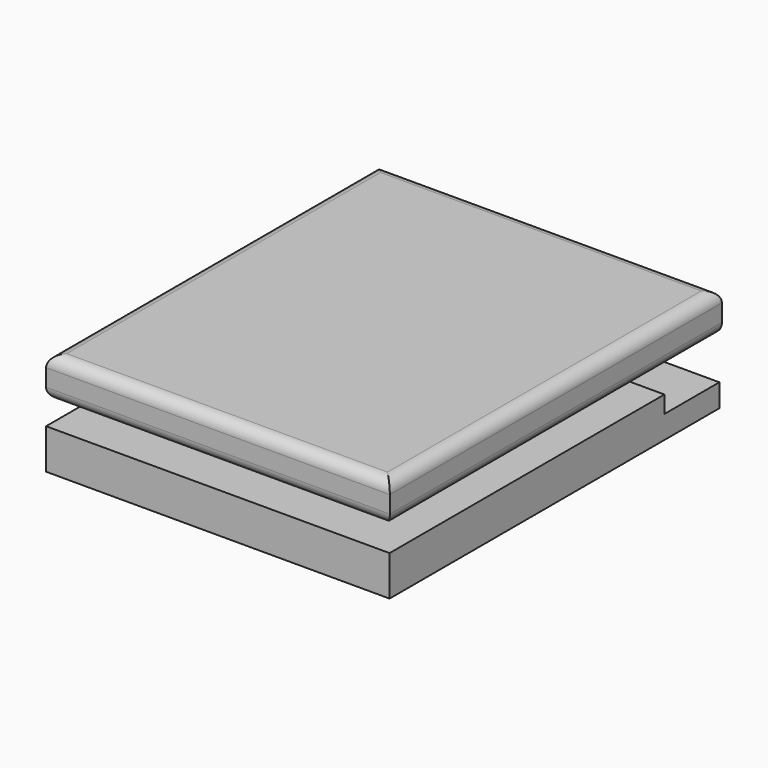
from build123d import *

# Parameters (mm, degrees)
F0_W        = 30
F0_H        = 30
F1_DEPTH    = 1.5
F2_W        = 15
F2_H        = 18.3394747698
F3_DEPTH    = 2
F4_W        = 30
F4_H        = 36
F5_DEPTH    = 2
F6_W        = 30.0186313689
F6_H        = 36.2569130957
F7_DEPTH    = 3.5
F8_T1_DEPTH = 15
F8_T3_DEPTH = 41.2569130957
F8_T5_DEPTH = 35.0186313689


# Not quite as in the source:
# - a fillet or chamfer that OpenCascade refuses, or shapes differently, is made with other operations: its cross-section is extruded or revolved along the edge and cut away or added


with BuildPart() as f1:
    # F0 (on Top) → F1 (new body)
    with BuildSketch(Plane.XY):
        with Locations((15, 15)):
            Rectangle(F0_W, F0_H)
    extrude(amount=F1_DEPTH)

    # F2 (on face) → F3 (join)
    with BuildSketch(Plane.XY.offset(1.5)):
        with Locations((14.8406922431, 27.8302626151)):
            Rectangle(F2_W, F2_H)
    extrude(amount=F3_DEPTH)

    # F4 (on face) → F5 (join)
    with BuildSketch(Plane(origin=(0, 0, 0), x_dir=(1, 0, 0), z_dir=(0, 0, -1))):
        with Locations((15, -18)):
            Rectangle(F4_W, F4_H)
    extrude(amount=F5_DEPTH)

    # F6 (on face) → F7 (join)
    with BuildSketch(Plane.XY.offset(3.5)):
        with Locations((15.0093156844, 18.1284565479)):
            Rectangle(F6_W, F6_H)
    extrude(amount=F7_DEPTH)

    # F8: fillet of radius 1 on 8 edges, made by hand

    # F8_s2 → F8_t1 (join)
    with BuildSketch(Plane.YZ.offset(7.3406922431)):
        with BuildLine():
            ThreePointArc((37, 3.5), (36.4641605821, 3.856890867), (36.2569130957, 4.4664345096))
            Line((36.2569130957, 4.4664345096), (36.2569130957, 3.5))
            Line((36.2569130957, 3.5), (37, 3.5))
        make_face()
    extrude(amount=F8_T1_DEPTH)

    # F8_s4 → F8_t3 (cut)
    with BuildSketch(Plane.XZ.offset(-38.7569130957)):
        with BuildLine():
            ThreePointArc((0, 6), (0.2928932188, 6.7071067812), (1, 7))
            Line((1, 7), (0, 7))
            Line((0, 7), (0, 6))
        make_face()
        with BuildLine():
            ThreePointArc((30.0186313689, 6), (29.7257381501, 6.7071067812), (29.0186313689, 7))
            Line((29.0186313689, 7), (30.0186313689, 7))
            Line((30.0186313689, 7), (30.0186313689, 6))
        make_face()
        with BuildLine():
            ThreePointArc((29.0186313689, 3.5), (29.7257381501, 3.7928932188), (30.0186313689, 4.5))
            Line((30.0186313689, 4.5), (30.0186313689, 3.5))
            Line((30.0186313689, 3.5), (29.0186313689, 3.5))
        make_face()
        with BuildLine():
            ThreePointArc((1, 3.5), (0.2928932188, 3.7928932188), (0, 4.5))
            Line((0, 4.5), (0, 3.5))
            Line((0, 3.5), (1, 3.5))
        make_face()
    extrude(amount=F8_T3_DEPTH, mode=Mode.SUBTRACT)

    # F8_s6 → F8_t5 (cut)
    with BuildSketch(Plane.YZ.offset(-2.5)):
        with BuildLine():
            ThreePointArc((36.2569130957, 6), (35.9640198769, 6.7071067812), (35.2569130957, 7))
            Line((35.2569130957, 7), (36.2569130957, 7))
            Line((36.2569130957, 7), (36.2569130957, 6))
        make_face()
        with BuildLine():
            ThreePointArc((0, 6), (0.2928932188, 6.7071067812), (1, 7))
            Line((1, 7), (0, 7))
            Line((0, 7), (0, 6))
        make_face()
        with BuildLine():
            ThreePointArc((1, 3.5), (0.2928932188, 3.7928932188), (0, 4.5))
            Line((0, 4.5), (0, 3.5))
            Line((0, 3.5), (1, 3.5))
        make_face()
    extrude(amount=F8_T5_DEPTH, mode=Mode.SUBTRACT)


solid = f1.part
